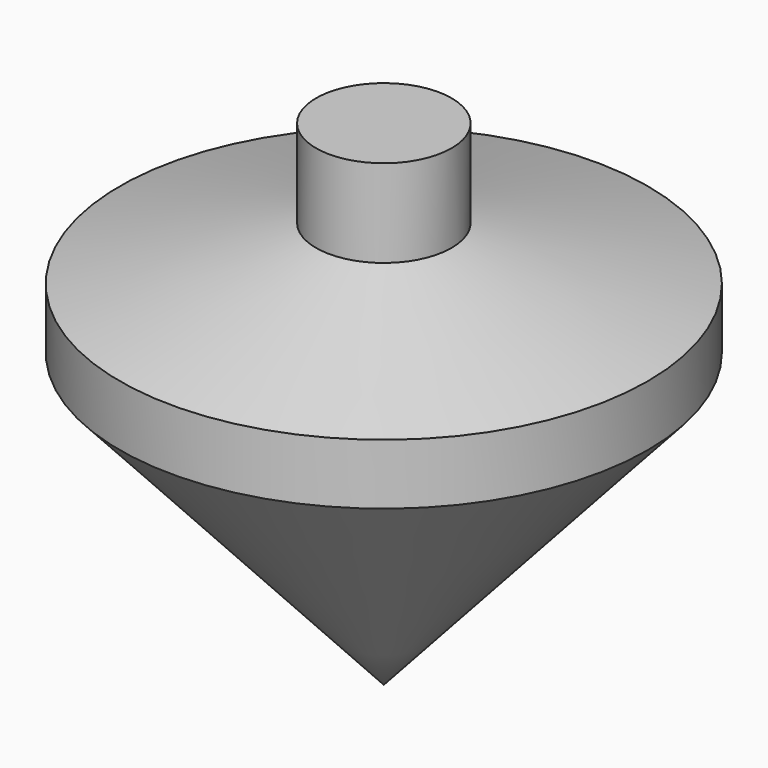
from build123d import *

# Parameters (mm, degrees)
F2_DEPTH = 6.35


# Not quite as in the source:
# - the program builds the solid bodies; features that only make, move or delete a surface that nothing else refers to are left out


with BuildPart() as f1:
    # F0 (on Front) → F1 (revolve)
    with BuildSketch(Plane.XZ):
        Polygon((0, 29.4230338186), (0, 0), (19.0991610289, 21.1639348418), (19.0991610289, 25.5515798926), (4.9038375728, 29.4230338186), align=None)
    revolve(axis=Axis((0, 0, 14.7115169093), (0, 0, -1)))

    # F2 (add): a face of the model
    f2_faces = [f1.faces().sort_by_distance(p)[0] for p in [
        (0, 0, 29.4230338186),
    ]]
    extrude(f2_faces, amount=F2_DEPTH)


solid = f1.part
